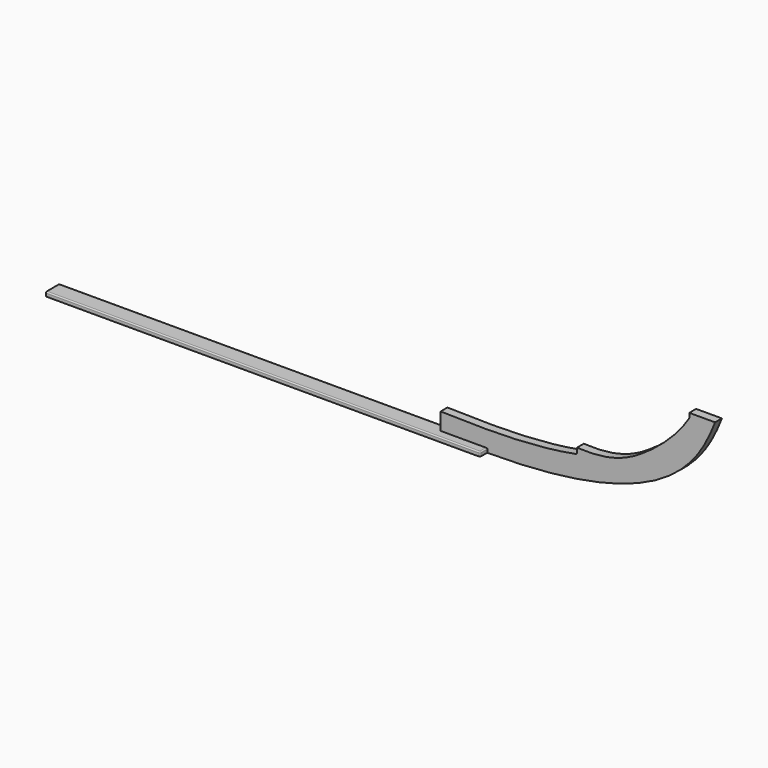
from build123d import *

# Parameters (mm, degrees)
F1_DEPTH = 38.1
F3_DEPTH = 76.2
F4_R     = 5.08
F5_R     = 5.08
F6_R     = 5.08


with BuildPart() as f1:
    # F0 (on Front) → F1 (new body)
    with BuildSketch(Plane.XZ):
        with BuildLine():
            add(Edge.make_bspline(
                [(-397.9034916449, -37.2863032911), (410.8181435335, -37.1667715246), (542.3002453184, 229.7381759582), (614.3201670874, 411.4448271791)],
                knots=[0, 0, 0, 0, 1107.2291374194, 1107.2291374194, 1107.2291374194, 1107.2291374194], degree=3))
            Line((614.3201670874, 411.4448271791), (499.5962828133, 411.4448271791))
            Line((499.5962828133, 411.4448271791), (499.5962828133, 390.5045126412))
            add(Edge.make_bspline(
                [(-0.08459932, 112.5677610649), (138.9812140865, 104.8921065828), (289.8373497184, 164.1537835287), (451.0105705046, 310.1172410619), (499.5962828133, 390.5045126412)],
                knots=[0, 0, 0, 0, 0.5062424529, 1, 1, 1, 1], degree=3))
            Line((-0.08459932, 112.5677610649), (-0.08459932, 91.3603947808))
            ThreePointArc((-0.08459932, 91.3603947808), (-1.2489795154, 88.1239891285), (-4.2083479602, 86.37120814))
            add(Edge.make_bspline(
                [(-606.6288212141, 57.1127695403), (-404.6368126357, 51.4652566588), (-200.4539536083, 48.7578373083), (-4.2083479602, 86.37120814)],
                knots=[0, 0, 0, 0, 603.0630991795, 603.0630991795, 603.0630991795, 603.0630991795], degree=3))
            Line((-606.6288212141, 57.1127695403), (-606.6288212141, -19.0872304597))
            Line((-606.6288212141, -19.0872304597), (-402.9834916449, -19.0872304597))
            ThreePointArc((-402.9834916449, -19.0872304597), (-399.3913891965, -20.5751280112), (-397.9034916449, -24.1672304597))
            Line((-397.9034916449, -24.1672304597), (-397.9034916449, -37.2863032911))
        make_face()
    extrude(amount=F1_DEPTH)


with BuildPart() as f3:
    # F2 (on Front) → F3 (new body)
    with BuildSketch(Plane.XZ):
        Polygon((-2330.9707720995, -38.3599539625), (-400.5707720995, -38.4839051044), (-400.5707720995, -19.4956134433), (-2330.9707720995, -19.4956134433), align=None)
    extrude(amount=F3_DEPTH)

    # F4
    f4_edges = [f3.edges().sort_by_distance(p)[0] for p in [
        (-400.570772, -38.1, -19.495613),
    ]]
    fillet(f4_edges, radius=F4_R)

    # F5
    f5_edges = [f3.edges().sort_by_distance(p)[0] for p in [
        (-1368.310772, -76.2, -19.495613),
    ]]
    fillet(f5_edges, radius=F5_R)

    # F6
    f6_edges = [f3.edges().sort_by_distance(p)[0] for p in [
        (-1368.310772, 0, -19.495613),
    ]]
    fillet(f6_edges, radius=F6_R)


solid = Compound([f1.part, f3.part])
